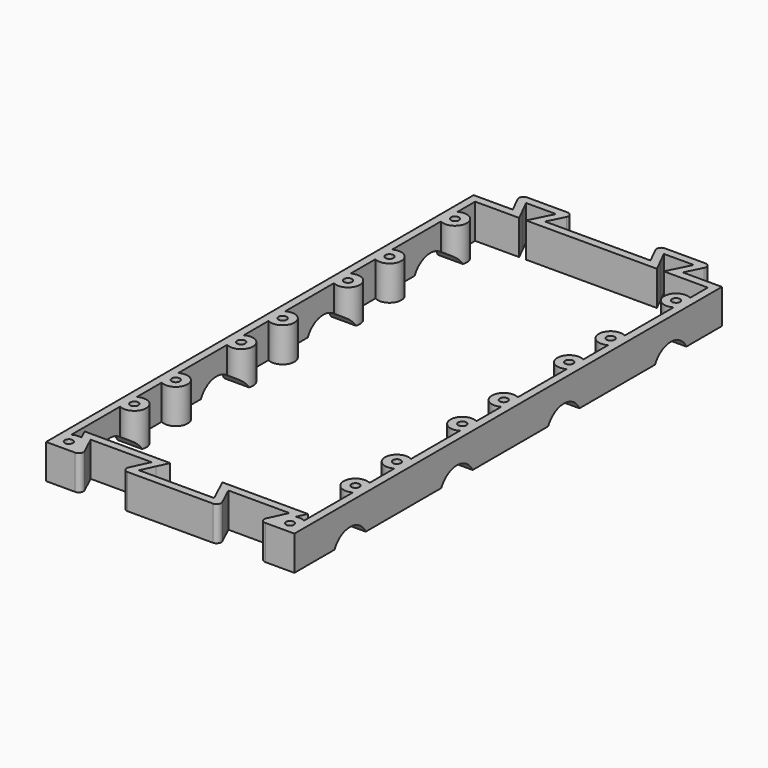
from build123d import *

# Parameters (mm, degrees)
F0_R        = 1.75
F1_DEPTH    = 15
F2_T        = 3.4
F2_T3_DEPTH = 21.8
F3_R        = 2
F5_DEPTH    = 200


# Not quite as in the source:
# - a shell that OpenCascade refuses in one call is made with other operations: the cavity is built on its own and cut out


with BuildPart() as f1:
    # F0 (on Top) → F1 (new body)
    with BuildSketch(Plane.XY):
        Polygon((17, 0), (0, 0), (0, -232), (15.75, -232), (10.75, -221.25), (37.25, -221.25), (32.25, -232), (75.55, -232), (70.55, -221.25), (97.05, -221.25), (92.05, -232), (107.8, -232), (107.8, 0), (90.8, 0), (95.8, 10), (71.8, 10), (76.8, 0), (31, 0), (36, 10), (12, 10), align=None)
        with Locations((5.9, -227)):
            Circle(F0_R, mode=Mode.SUBTRACT)
        with Locations((5.9, -191.5)):
            Circle(F0_R, mode=Mode.SUBTRACT)
        with Locations((5.9, -169)):
            Circle(F0_R, mode=Mode.SUBTRACT)
        with Locations((5.9, -133.5)):
            Circle(F0_R, mode=Mode.SUBTRACT)
        with Locations((101.9, -227)):
            Circle(F0_R, mode=Mode.SUBTRACT)
        with Locations((101.9, -191.5)):
            Circle(F0_R, mode=Mode.SUBTRACT)
        with Locations((101.9, -169)):
            Circle(F0_R, mode=Mode.SUBTRACT)
        with Locations((101.9, -133.5)):
            Circle(F0_R, mode=Mode.SUBTRACT)
        with Locations((5.9, -111)):
            Circle(F0_R, mode=Mode.SUBTRACT)
        with Locations((5.9, -75.5)):
            Circle(F0_R, mode=Mode.SUBTRACT)
        with Locations((5.9, -53)):
            Circle(F0_R, mode=Mode.SUBTRACT)
        with Locations((5.9, -17.5)):
            Circle(F0_R, mode=Mode.SUBTRACT)
        with Locations((101.9, -111)):
            Circle(F0_R, mode=Mode.SUBTRACT)
        with Locations((101.9, -75.5)):
            Circle(F0_R, mode=Mode.SUBTRACT)
        with Locations((101.9, -53)):
            Circle(F0_R, mode=Mode.SUBTRACT)
        with Locations((101.9, -17.5)):
            Circle(F0_R, mode=Mode.SUBTRACT)
    extrude(amount=F1_DEPTH)

    # F2: shell of thickness 3.4, made by hand


with BuildPart() as f2_core1:
    # F2_t2: copy of F1
    add(f1.part)

    # the walls: a layer under each face that stays
    f2_faces = [f2_core1.faces().sort_by_distance(p)[0] for p in [
        (8.5, 0, 7.5),
        (0, -116, 7.5),
        (7.875, -232, 7.5),
        (13.25, -226.625, 7.5),
        (24, -221.25, 7.5),
        (34.75, -226.625, 7.5),
        (53.9, -232, 7.5),
        (73.05, -226.625, 7.5),
        (83.8, -221.25, 7.5),
        (94.55, -226.625, 7.5),
        (99.925, -232, 7.5),
        (107.8, -116, 7.5),
        (99.3, 0, 7.5),
        (93.3, 5, 7.5),
        (83.8, 10, 7.5),
        (74.3, 5, 7.5),
        (53.9, 0, 7.5),
        (33.5, 5, 7.5),
        (24, 10, 7.5),
        (14.5, 5, 7.5),
        (4.15, -227, 7.5),
        (4.15, -191.5, 7.5),
        (4.15, -169, 7.5),
        (4.15, -133.5, 7.5),
        (100.15, -227, 7.5),
        (100.15, -191.5, 7.5),
        (100.15, -169, 7.5),
        (100.15, -133.5, 7.5),
        (4.15, -111, 7.5),
        (4.15, -75.5, 7.5),
        (4.15, -53, 7.5),
        (4.15, -17.5, 7.5),
        (100.15, -111, 7.5),
        (100.15, -75.5, 7.5),
        (100.15, -53, 7.5),
        (100.15, -17.5, 7.5),
    ]]
    thicken(f2_faces, amount=-F2_T, mode=Mode.SUBTRACT)

    # F2_s4 → F2_t3 (cut)
    with BuildSketch(Plane.XY.offset(-3.4)):
        Polygon((16.9695894755, 0.0187947378), (17, -3.4), (22.5013155617, -3.4), (20.0410524494, 1.5205262247), align=None)
        Polygon((10.7808285178, -221.2696611545), (7.6671482196, -222.683884549), (5.4188298247, -217.85), (10.75, -217.85), align=None)
        Polygon((37.2191714822, -221.2696611545), (37.25, -217.85), (42.5811701753, -217.85), (40.3328517804, -222.683884549), align=None)
        Polygon((70.5808285178, -221.2696611545), (67.4671482196, -222.683884549), (65.2188298247, -217.85), (70.55, -217.85), align=None)
        Polygon((97.0191714822, -221.2696611545), (97.05, -217.85), (102.3811701753, -217.85), (100.1328517804, -222.683884549), align=None)
        Polygon((90.8304105245, 0.0187947378), (90.8, -3.4), (85.2986844383, -3.4), (87.7589475506, 1.5205262247), align=None)
        Polygon((76.7695894755, 0.0187947378), (79.8410524494, 1.5205262247), (82.3013155617, -3.4), (76.8, -3.4), align=None)
        Polygon((31.0304105245, 0.0187947378), (31, -3.4), (25.4986844383, -3.4), (27.9589475506, 1.5205262247), align=None)
    extrude(amount=F2_T3_DEPTH, mode=Mode.SUBTRACT)


with BuildPart() as f1_1:
    add(f1.part)

    # what is left inside the walls is the cavity
    f2_cavity = [f2_core1.part.solids().sort_by_distance(p)[0] for p in [
        (53.9, -150.2, 14.966),
    ]]
    add(f2_cavity, mode=Mode.SUBTRACT)

    # F3
    f3_edges = [f1_1.edges().sort_by_distance(p)[0] for p in [
        (15.75, -232, 7.5),
        (32.25, -232, 7.5),
        (75.55, -232, 7.5),
        (92.05, -232, 7.5),
        (12, 10, 7.5),
        (36, 10, 7.5),
        (71.8, 10, 7.5),
        (95.8, 10, 7.5),
    ]]
    fillet(f3_edges, radius=F3_R)

    # F4 (on face) → F5 (cut)
    with BuildSketch(Plane.YZ.offset(107.8)):
        with BuildLine():
            Line((-210.2734148502, 0), (-193.2988762856, 0))
            ThreePointArc((-193.2988762856, 0), (-201.7861455679, 5.2826077701), (-210.2734148502, 0))
        make_face()
        with BuildLine():
            ThreePointArc((-135.2988762856, 0), (-143.7861455679, 5.2826077701), (-152.2734148502, 0))
            Line((-152.2734148502, 0), (-135.2988762856, 0))
        make_face()
        with BuildLine():
            ThreePointArc((-77.2988762856, 0), (-85.7861455679, 5.2826077701), (-94.2734148502, 0))
            Line((-94.2734148502, 0), (-77.2988762856, 0))
        make_face()
        with BuildLine():
            ThreePointArc((-19.2988762856, 0), (-27.7861455679, 5.2826077701), (-36.2734148502, 0))
            Line((-36.2734148502, 0), (-19.2988762856, 0))
        make_face()
    extrude(amount=-F5_DEPTH, mode=Mode.SUBTRACT)


solid = f1_1.part
